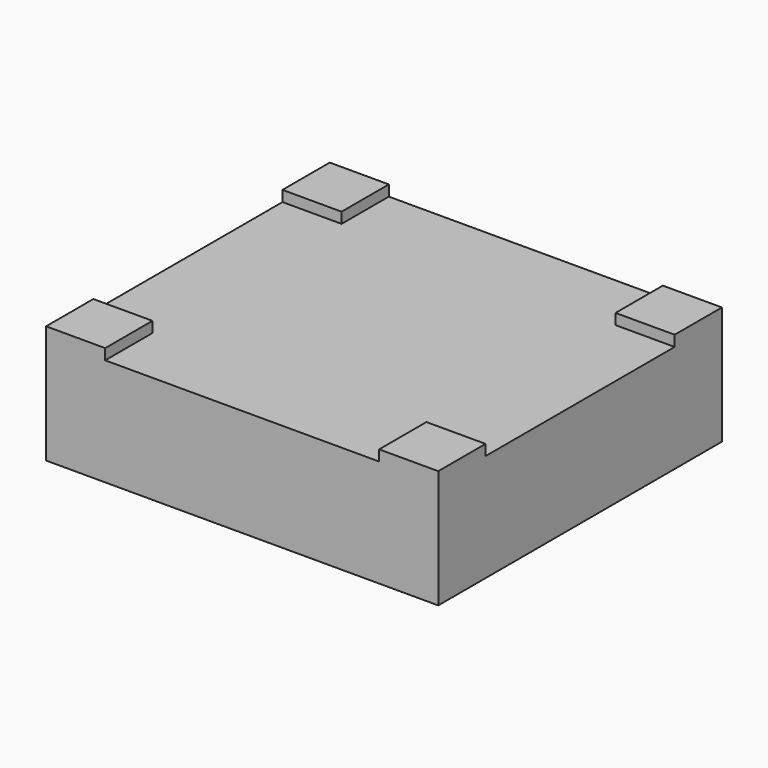
from build123d import *

# Parameters (mm, degrees)
F0_W     = 115.8875
F0_H     = 104.775
F1_DEPTH = 31.75
F2_W     = 17.4625
F2_H     = 17.4625
F3_DEPTH = 3.175


# Not quite as in the source:
# - a length typed as a fraction of an inch, garbled in the dataset ("3 / 203.2 mm" for 3/8 in), is restored


with BuildPart() as f1:
    # F0 (on Top) → F1 (new body)
    with BuildSketch(Plane.XY):
        with Locations((0.44375, -0.3875)):
            Rectangle(F0_W, F0_H)
    extrude(amount=F1_DEPTH)

    # F2 (on face) → F3 (join)
    with BuildSketch(Plane.XY.offset(31.75)):
        with Locations((-48.76875, 43.26875)):
            Rectangle(F2_W, F2_H)
        with Locations((49.65625, 43.26875)):
            Rectangle(F2_W, F2_H)
        with Locations((-48.76875, -44.04375)):
            Rectangle(F2_W, F2_H)
        with Locations((49.65625, -44.04375)):
            Rectangle(F2_W, F2_H)
    extrude(amount=F3_DEPTH)


solid = f1.part
